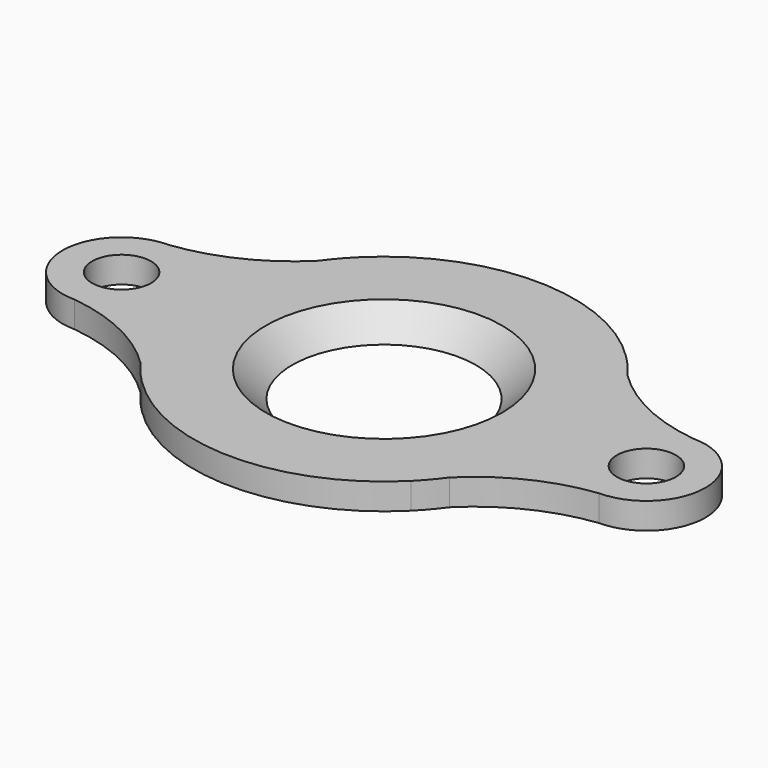
from build123d import *

# Parameters (mm, degrees)
F0_R     = 7
F0_R_2   = 2.25
F1_DEPTH = 2
F2_SIZE  = 1.99999


# Not quite as in the source:
# - a fillet or chamfer is up to 0.001 mm smaller than in the source, because OpenCascade refuses the exact size


with BuildPart() as f1:
    # F0 (on Top) → F1 (new body)
    with BuildSketch(Plane.XY):
        with BuildLine():
            ThreePointArc((11.7645575334, 8.4761539653), (10.9717281133, 9.333063578), (10.2530483272, 10.2530483272))
            ThreePointArc((10.2530483272, 10.2530483272), (0, 14.5), (-10.2530483272, 10.2530483272))
            ThreePointArc((-10.2530483272, 10.2530483272), (-10.9717281133, 9.333063578), (-11.7645575334, 8.4761539653))
            ThreePointArc((-11.7645575334, 8.4761539653), (-14.5, 0), (-11.7645575334, -8.4761539653))
            ThreePointArc((-11.7645575334, -8.4761539653), (-10.9717281133, -9.333063578), (-10.2530483272, -10.2530483272))
            ThreePointArc((-10.2530483272, -10.2530483272), (0, -14.5), (10.2530483272, -10.2530483272))
            ThreePointArc((10.2530483272, -10.2530483272), (10.9717281133, -9.333063578), (11.7645575334, -8.4761539653))
            ThreePointArc((11.7645575334, -8.4761539653), (13.7992044016, -4.4533086445), (14.5, 0))
            ThreePointArc((14.5, 0), (13.7992044016, 4.4533086445), (11.7645575334, 8.4761539653))
        make_face()
        Circle(F0_R, mode=Mode.SUBTRACT)
        with BuildLine():
            ThreePointArc((11.7645575334, 8.4761539653), (11.0445950741, 9.3950476129), (10.2530483272, 10.2530483272))
            ThreePointArc((10.2530483272, 10.2530483272), (10.9717281133, 9.333063578), (11.7645575334, 8.4761539653))
        make_face()
        with BuildLine():
            ThreePointArc((-11.7645575334, 8.4761539653), (-10.9717281133, 9.333063578), (-10.2530483272, 10.2530483272))
            ThreePointArc((-10.2530483272, 10.2530483272), (-11.0445950741, 9.3950476129), (-11.7645575334, 8.4761539653))
        make_face()
        with BuildLine():
            ThreePointArc((20, 4.5), (15.5484628484, 5.7966747348), (11.7645575334, 8.4761539653))
            ThreePointArc((11.7645575334, 8.4761539653), (13.7992044016, 4.4533086445), (14.5, 0))
            ThreePointArc((14.5, 0), (13.7992044016, -4.4533086445), (11.7645575334, -8.4761539653))
            ThreePointArc((11.7645575334, -8.4761539653), (15.5484628484, -5.7966747348), (20, -4.5))
            ThreePointArc((20, -4.5), (24.5, 0), (20, 4.5))
        make_face()
        with Locations((20, 0)):
            Circle(F0_R_2, mode=Mode.SUBTRACT)
        with BuildLine():
            ThreePointArc((-11.7645575334, -8.4761539653), (-14.5, 0), (-11.7645575334, 8.4761539653))
            ThreePointArc((-11.7645575334, 8.4761539653), (-15.5484628484, 5.7966747348), (-20, 4.5))
            ThreePointArc((-20, 4.5), (-24.5, 0), (-20, -4.5))
            ThreePointArc((-20, -4.5), (-15.5484628484, -5.7966747348), (-11.7645575334, -8.4761539653))
        make_face()
        with Locations((-20, 0)):
            Circle(F0_R_2, mode=Mode.SUBTRACT)
        with BuildLine():
            ThreePointArc((-10.2530483272, -10.2530483272), (-10.9717281133, -9.333063578), (-11.7645575334, -8.4761539653))
            ThreePointArc((-11.7645575334, -8.4761539653), (-11.0445950741, -9.3950476129), (-10.2530483272, -10.2530483272))
        make_face()
        with BuildLine():
            ThreePointArc((10.2530483272, -10.2530483272), (11.0445950741, -9.3950476129), (11.7645575334, -8.4761539653))
            ThreePointArc((11.7645575334, -8.4761539653), (10.9717281133, -9.333063578), (10.2530483272, -10.2530483272))
        make_face()
    extrude(amount=F1_DEPTH)

    # F2 (size 2 in the source; OpenCascade refuses exactly that, so slightly less here)
    f2_edges = [f1.edges().sort_by_distance(p)[0] for p in [
        (-7, 0, 2),
    ]]
    chamfer(f2_edges, length=F2_SIZE)


solid = f1.part
